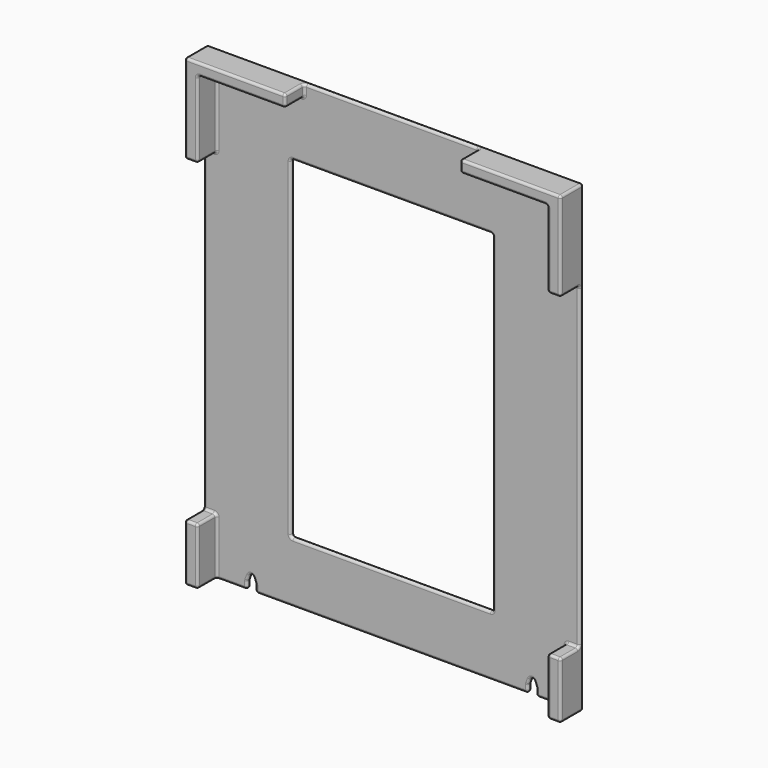
from build123d import *

# Parameters (mm, degrees)
F0_W     = 5.5
F0_H     = 23.9701914787
F1_DEPTH = 2
F2_DEPTH = 12
F3_W     = 85
F3_H     = 140
F4_DEPTH = 25
F5_R     = 0.99999


# Not quite as in the source:
# - a fillet or chamfer is up to 0.001 mm smaller than in the source, because OpenCascade refuses the exact size


with BuildPart() as f1:
    # F0 (on Front) → F1 (new body)
    with BuildSketch(Plane.XZ):
        with BuildLine():
            Line((-36.75, 185), (-73.5, 185))
            Line((-73.5, 185), (-73.5, 152.6025086641))
            Line((-73.5, 152.6025086641), (-79, 152.6025086641))
            Line((-79, 152.6025086641), (-79, 18.9701914787))
            Line((-79, 18.9701914787), (-73.5, 18.9701914787))
            Line((-73.5, 18.9701914787), (-73.5, -5))
            Line((-73.5, -5), (-60.75, -5))
            Line((-60.75, -5), (-60.75, -1.8105786294))
            Line((-60.75, -1.8105786294), (-59.9358969391, 0.3522739267))
            ThreePointArc((-59.9358969391, 0.3522739267), (-59, 1), (-58.0641030609, 0.3522739267))
            Line((-58.0641030609, 0.3522739267), (-57.25, -1.8105786294))
            Line((-57.25, -1.8105786294), (-57.25, -5))
            Line((-57.25, -5), (0, -5))
            Line((0, -5), (57.25, -5))
            Line((57.25, -5), (57.25, -1.8105786294))
            Line((57.25, -1.8105786294), (58.0641030609, 0.3522739267))
            ThreePointArc((58.0641030609, 0.3522739267), (59, 1), (59.9358969391, 0.3522739267))
            Line((59.9358969391, 0.3522739267), (60.75, -1.8105786294))
            Line((60.75, -1.8105786294), (60.75, -5))
            Line((60.75, -5), (73.5, -5))
            Line((73.5, -5), (73.5, 18.9701914787))
            Line((73.5, 18.9701914787), (79, 18.9701914787))
            Line((79, 18.9701914787), (79, 152.6025086641))
            Line((79, 152.6025086641), (73.5, 152.6025086641))
            Line((73.5, 152.6025086641), (73.5, 185))
            Line((73.5, 185), (36.75, 185))
            Line((36.75, 185), (36.75, 190))
            Line((36.75, 190), (0, 190))
            Line((0, 190), (-36.75, 190))
            Line((-36.75, 190), (-36.75, 185))
        make_face()
        Polygon((-73.5, 152.6025086641), (-73.5, 185), (-36.75, 185), (-36.75, 190), (-79, 190), (-79, 152.6025086641), align=None)
        Polygon((79, 190), (36.75, 190), (36.75, 185), (73.5, 185), (73.5, 152.6025086641), (79, 152.6025086641), align=None)
        with Locations((76.25, 6.9850957394)):
            Rectangle(F0_W, F0_H)
        with Locations((-76.25, 6.9850957394)):
            Rectangle(F0_W, F0_H)
    extrude(amount=F1_DEPTH)

    # F0 (on Front) → F2 (join)
    with BuildSketch(Plane.XZ):
        Polygon((79, 190), (36.75, 190), (36.75, 185), (73.5, 185), (73.5, 152.6025086641), (79, 152.6025086641), align=None)
        Polygon((-73.5, 152.6025086641), (-73.5, 185), (-36.75, 185), (-36.75, 190), (-79, 190), (-79, 152.6025086641), align=None)
        with Locations((-76.25, 6.9850957394)):
            Rectangle(F0_W, F0_H)
        with Locations((76.25, 6.9850957394)):
            Rectangle(F0_W, F0_H)
    extrude(amount=F2_DEPTH)

    # F3 (on face) → F4 (cut)
    with BuildSketch(Plane.XZ.offset(2)):
        with Locations((0, 90.2203150839)):
            Rectangle(F3_W, F3_H)
    extrude(amount=-F4_DEPTH, mode=Mode.SUBTRACT)

    # F5 (radius 1 in the source; OpenCascade refuses exactly that, so slightly less here)
    f5_edges = [f1.edges().sort_by_distance(p)[0] for p in [
        (55.125, -12, 185),
        (-73.5, -12, 168.801254),
        (0, -2, 20.220315),
        (-57.875, -12, 190),
        (57.875, -12, 190),
        (73.5, -12, 6.985096),
        (-79, -12, 171.301254),
        (36.75, -12, 187.5),
        (-73.5, -12, 6.985096),
        (76.25, -12, 18.970191),
        (60.75, -2, -3.405289),
        (-76.25, -12, -5),
        (-60.75, -1, -5),
        (73.5, -7, 185),
        (-57.25, -2, -3.405289),
        (0, -2, -5),
        (-76.25, -12, 18.970191),
        (-55.125, -12, 185),
        (79, -12, 171.301254),
        (73.5, -12, 168.801254),
        (79, -2, 85.78635),
        (-79, -12, 6.985096),
        (0, -2, 190),
        (-79, -2, 85.78635),
        (76.25, -12, -5),
        (-67.125, -2, -5),
        (67.125, -2, -5),
        (-76.25, -12, 152.602509),
        (79, -12, 6.985096),
        (-42.5, -1, 20.220315),
        (42.5, -1, 20.220315),
        (0, -2, 160.220315),
        (-42.5, -2, 90.220315),
        (42.5, -2, 90.220315),
        (-57.657052, -2, -0.729152),
        (-57.25, -1, -5),
        (-57.25, 0, -3.405289),
        (0, 0, -5),
        (-60.75, -2, -3.405289),
        (59, -2, 1),
        (-60.342948, -2, -0.729152),
        (60.75, -1, -5),
        (60.75, -1, -1.810579),
        (60.342948, -2, -0.729152),
        (-57.25, -1, -1.810579),
        (55.125, -2, 185),
        (36.75, -7, 185),
        (-73.5, -7, -5),
        (-59, -2, 1),
        (-55.125, -2, 185),
        (57.25, -2, -3.405289),
        (57.657052, -2, -0.729152),
        (-36.75, -12, 187.5),
        (73.5, -2, 6.985096),
        (36.75, -7, 190),
        (-73.5, -2, 168.801254),
        (-79, -7, 152.602509),
        (-73.5, -7, 185),
        (-76.25, -2, 18.970191),
        (-79, -6, 190),
        (-79, -6, -5),
        (79, -6, -5),
        (79, -6, 190),
        (0, 0, 190),
        (76.25, -12, 152.602509),
        (-79, 0, 92.5),
        (-69.875, 0, -5),
        (69.875, 0, -5),
        (79, 0, 92.5),
        (73.5, -7, 18.970191),
        (-73.5, -7, 18.970191),
        (79, -7, 18.970191),
        (73.5, -2, 168.801254),
        (-79, -7, 18.970191),
        (73.5, -7, -5),
        (-73.5, -7, 152.602509),
        (42.5, -1, 160.220315),
        (0, 0, 160.220315),
        (0, 0, 20.220315),
        (42.5, 0, 90.220315),
        (-42.5, -1, 160.220315),
        (58.064103, -1, 0.352274),
        (57.25, 0, -3.405289),
        (-60.75, -1, -1.810579),
        (57.25, -1, -1.810579),
        (60.342948, 0, -0.729152),
        (59.935897, -1, 0.352274),
        (-60.75, 0, -3.405289),
        (-58.064103, -1, 0.352274),
        (-59.935897, -1, 0.352274),
        (57.657052, 0, -0.729152),
        (-57.657052, 0, -0.729152),
        (57.25, -1, -5),
        (-60.342948, 0, -0.729152),
        (60.75, 0, -3.405289),
        (36.75, -2, 187.5),
        (-36.75, -7, 190),
        (-76.25, -2, 152.602509),
        (73.5, -7, 152.602509),
        (76.25, -2, 18.970191),
        (-36.75, -7, 185),
        (-73.5, -2, 6.985096),
        (-36.75, -2, 187.5),
        (79, -7, 152.602509),
        (76.25, -2, 152.602509),
        (-42.5, 0, 90.220315),
        (-59, 0, 1),
        (59, 0, 1),
    ]]
    fillet(f5_edges, radius=F5_R)


solid = f1.part
